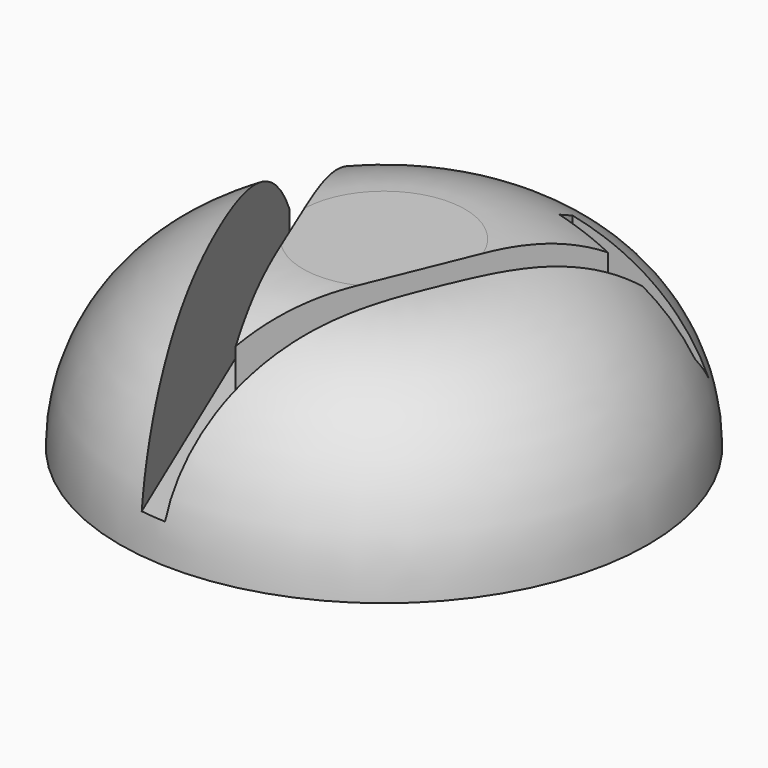
from build123d import *

# Parameters (mm, degrees)
F0_R         = 36.0587113204
F1_DEPTH     = 25
F2_R         = 24.99999
F3_TEXT_SIZE = 87.0668355169
F4_DEPTH     = 20


# Not quite as in the source:
# - a fillet or chamfer is up to 0.001 mm smaller than in the source, because OpenCascade refuses the exact size
# - Text() gives the source's letters only with a copy of the font that has no kerning and outlines rounded to 1/6400 em; it was checked with that copy


with BuildPart() as f1:
    # F0 (on Top) → F1 (new body)
    with BuildSketch(Plane.XY):
        Circle(F0_R)
    extrude(amount=F1_DEPTH)

    # F2 (radius 25 in the source; OpenCascade refuses exactly that, so slightly less here)
    f2_edges = [f1.edges().sort_by_distance(p)[0] for p in [
        (-36.058711, 0, 25),
    ]]
    fillet(f2_edges, radius=F2_R)

    # F3 (on face) → F4 (cut)
    with BuildSketch(Plane.XY.offset(25)):
        with Locations((-34.7747541964, -35.5544574559)):
            Text('V', F3_TEXT_SIZE, font='Tinos', text_align=(TextAlign.LEFT, TextAlign.BOTTOM))
    extrude(amount=-F4_DEPTH, mode=Mode.SUBTRACT)


solid = f1.part
